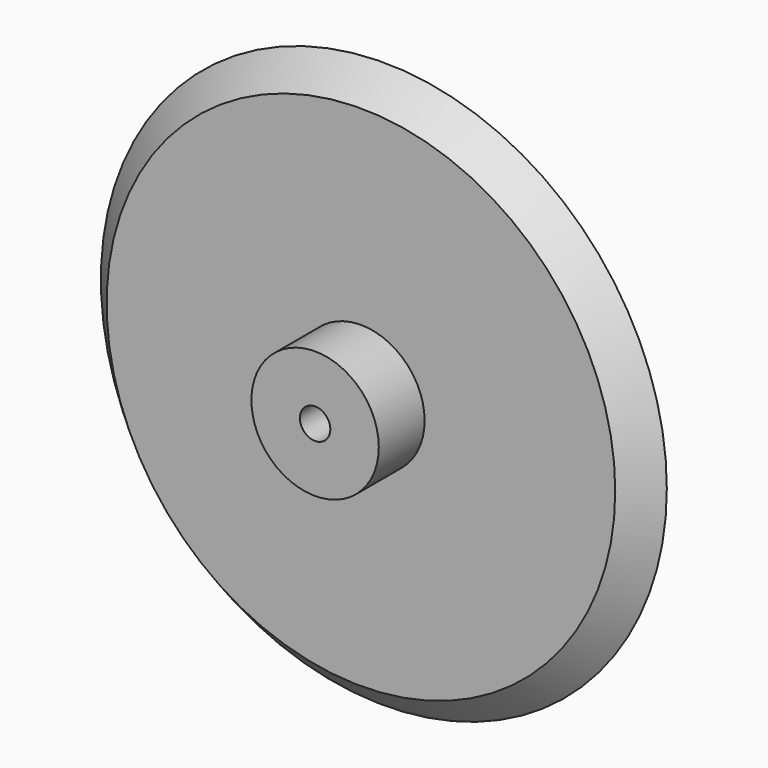
from build123d import *

# Parameters (mm, degrees)
F0_R     = 22.75
F1_DEPTH = 2
F2_R     = 4.4458772924
F3_DEPTH = 6
F4_R     = 4.4949655375
F5_DEPTH = 3
F6_R     = 1.0635
F7_DEPTH = 6
F8_R     = 1.0635
F9_DEPTH = 6


# Not quite as in the source:
# - a fillet or chamfer that OpenCascade refuses, or shapes differently, is made with other operations: its cross-section is extruded or revolved along the edge and cut away or added


with BuildPart() as f1:
    # F0 (on Front) → F1 (new body)
    with BuildSketch(Plane.XZ):
        Circle(F0_R)
    extrude(amount=F1_DEPTH)

    # F2 (on Front) → F3 (join)
    with BuildSketch(Plane.XZ):
        Circle(F2_R)
    extrude(amount=F3_DEPTH)

    # F4 (on Front) → F5 (join)
    with BuildSketch(Plane.XZ):
        Circle(F4_R)
    extrude(amount=-F5_DEPTH)

    # F6 (on Front) → F7 (cut)
    with BuildSketch(Plane.XZ):
        Circle(F6_R)
    extrude(amount=F7_DEPTH, mode=Mode.SUBTRACT)

    # F8 (on Front) → F9 (cut)
    with BuildSketch(Plane.XZ):
        Circle(F8_R)
    extrude(amount=-F9_DEPTH, mode=Mode.SUBTRACT)

    # F10: chamfer of 5 on 1 edges, made by hand

    # F10_s1 → F10_t2 (revolve, cut)
    with BuildSketch(Plane.XY):
        Polygon((22.75, 3), (17.75, -2), (22.75, -2), align=None)
    revolve(axis=Axis((0, -2, 0), (0, -1, 0)), mode=Mode.SUBTRACT)


solid = f1.part
